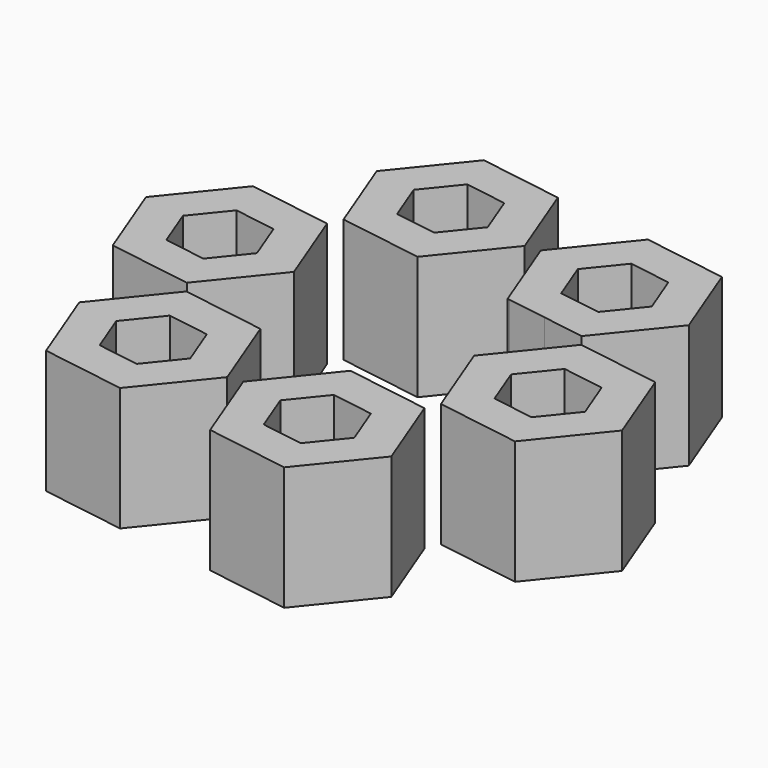
from build123d import *

# Parameters (mm, degrees)
F1_DEPTH = 25.4


with BuildPart() as f1:
    # F0 (on Top) → F1 (new body)
    with BuildSketch(Plane.XY):
        Polygon((-72.0923932347, -38.7846963805), (-54.7084513345, -41.518807573), (-43.648670635, -27.8309278658), (-49.9728318356, -11.4089369661), (-67.3567737358, -8.6748257736), (-78.4165544353, -22.3627054808), align=None)
        Polygon((-55.5027221854, -18.2528768197), (-52.3406415851, -26.4638722695), (-57.8705319349, -33.3078121231), (-66.5625028849, -31.9407565269), (-69.7245834852, -23.7297610771), (-64.1946931355, -16.8858212235), align=None, mode=Mode.SUBTRACT)
    extrude(amount=F1_DEPTH)


with BuildPart() as f1b:
    # F0 (on Top) → F1, piece 2 (new body)
    with BuildSketch(Plane.XY):
        Polygon((-55.1450750988, 7.8043004941), (-48.8209138982, -8.6176904056), (-31.436971998, -11.3518015981), (-20.3771912985, 2.3360781091), (-26.7013524991, 18.7580690088), (-44.0852943993, 21.4921802013), align=None)
        Polygon((-29.0691622486, 3.7031337054), (-34.5990525983, -3.1408061482), (-43.2910235484, -1.773750552), (-46.4531041487, 6.4372448978), (-40.9232137989, 13.2811847514), (-32.2312428489, 11.9141291552), align=None, mode=Mode.SUBTRACT)
    extrude(amount=F1_DEPTH)


with BuildPart() as f1c:
    # F0 (on Top) → F1, piece 3 (new body)
    with BuildSketch(Plane.XY):
        Polygon((-5.3066483048, -6.8790509105), (-10.6132966097, -13.758101821), (-2.3678097495, -15.0549353034), (-1.1839048747, -7.5274676517), align=None)
        Polygon((-6.3241612006, 16.4219908997), (-17.3839419001, 2.7341111925), (-11.0597806995, -13.6878797072), (-10.6132966097, -13.758101821), (-5.3066483048, -6.8790509105), (-5.5298903498, -6.8439398536), (-8.6919709501, 1.3670555962), (-3.1620806003, 8.2109954498), (5.5298903498, 6.8439398536), (8.6919709501, -1.3670555962), (3.1620806003, -8.2109954498), (-1.1839048747, -7.5274676517), (-2.3678097495, -15.0549353034), (6.3241612006, -16.4219908997), (17.3839419001, -2.7341111925), (11.0597806995, 13.6878797072), align=None)
    extrude(amount=F1_DEPTH)


with BuildPart() as f1d:
    # F0 (on Top) → F1, piece 4 (new body)
    with BuildSketch(Plane.XY):
        Polygon((25.5494345617, -21.5493155693), (8.1654926615, -18.8152043769), (-2.894288038, -32.503084084), (3.4298731626, -48.9250749837), (20.8138150627, -51.6591861762), (31.8735957623, -37.971306469), align=None)
        Polygon((8.9597635124, -42.0811351301), (5.7976829121, -33.8701396803), (11.3275732618, -27.0261998267), (20.0195442119, -28.3932554229), (23.1816248122, -36.6042508728), (17.6517344624, -43.4481907264), align=None, mode=Mode.SUBTRACT)
    extrude(amount=F1_DEPTH)


with BuildPart() as f1e:
    # F0 (on Top) → F1, piece 5 (new body)
    with BuildSketch(Plane.XY):
        Polygon((8.6021164258, -68.1383124439), (2.2779552252, -51.7163215442), (-15.105986675, -48.9822103518), (-26.1657673745, -62.670090059), (-19.8416061739, -79.0920809586), (-2.4576642738, -81.8261921511), align=None)
        Polygon((-17.4737964244, -64.0371456552), (-11.9439060747, -57.1932058016), (-3.2519351246, -58.5602613978), (-0.0898545243, -66.7712568477), (-5.6197448741, -73.6151967013), (-14.3117158241, -72.248141105), align=None, mode=Mode.SUBTRACT)
    extrude(amount=F1_DEPTH)


with BuildPart() as f1f:
    # F0 (on Top) → F1, piece 6 (new body)
    with BuildSketch(Plane.XY):
        Polygon((-40.2187974724, -76.7560028495), (-29.1590167729, -63.0681231423), (-35.4831779735, -46.6461322426), (-52.8671198736, -43.9120210502), (-63.9269005732, -57.5999007573), (-57.6027393725, -74.021891657), align=None)
        Polygon((-49.7050392733, -52.1230165), (-41.0130683233, -53.4900720962), (-37.850987723, -61.7010675461), (-43.3808780727, -68.5450073997), (-52.0728490228, -67.1779518034), (-55.2349296231, -58.9669563536), align=None, mode=Mode.SUBTRACT)
    extrude(amount=F1_DEPTH)


solid = Compound([f1.part, f1b.part, f1c.part, f1d.part, f1e.part, f1f.part])
